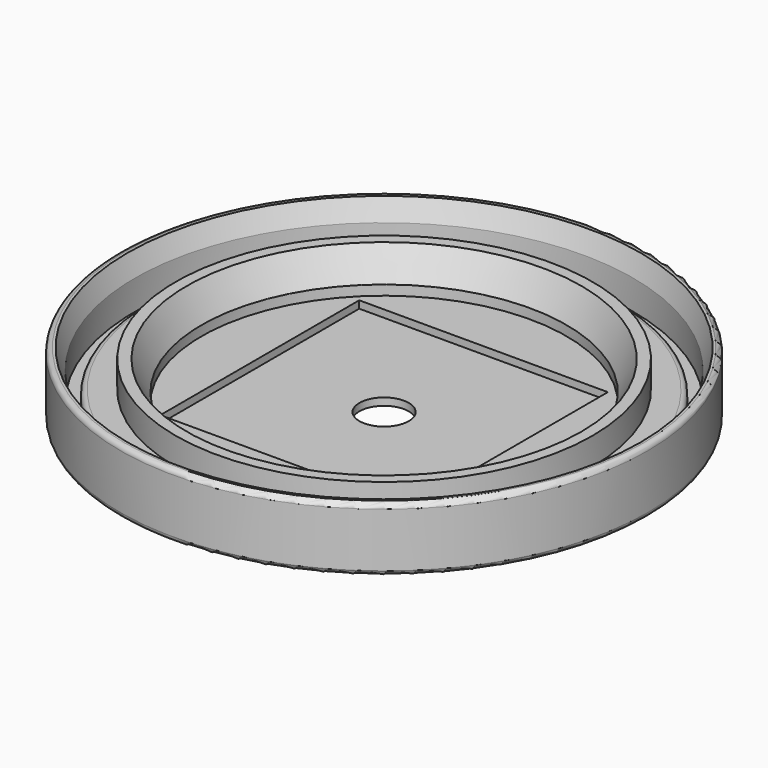
from build123d import *

# Parameters (mm, degrees)
F0_R      = 53.5
F1_DEPTH  = 13
F2_T      = -3
F3_R      = 48
F3_R_2    = 42.25
F3_R_3    = 37
F4_DEPTH  = 2.5
F5_DEPTH  = 8
F6_SIZE2  = 6
F6_SIZE   = 3
F7_SIZE2  = 1.5
F7_SIZE   = 4
F8_R      = 1
F9_R      = 5
F10_DEPTH = 45.7
F11_W     = 50.4
F11_H     = 50.4
F12_DEPTH = 1.5


with BuildPart() as f1:
    # F0 (on Top) → F1 (new body)
    with BuildSketch(Plane.XY):
        Circle(F0_R)
    extrude(amount=F1_DEPTH)

    # F2
    f2_openings = [f1.faces().sort_by_distance(p)[0] for p in [
        (0, 0, 13),
    ]]
    offset(amount=F2_T, openings=f2_openings)

    # F3 (on face) → F4 (join)
    with BuildSketch(Plane.XY.offset(3)):
        Circle(F3_R)
        Circle(F3_R_2, mode=Mode.SUBTRACT)
        Circle(F3_R_2)
        Circle(F3_R_3, mode=Mode.SUBTRACT)
    extrude(amount=F4_DEPTH)

    # F3 (on face) → F5 (join)
    with BuildSketch(Plane.XY.offset(3)):
        Circle(F3_R_2)
        Circle(F3_R_3, mode=Mode.SUBTRACT)
    extrude(amount=F5_DEPTH)

    # F6
    f6_edges = [f1.edges().sort_by_distance(p)[0] for p in [
        (-37, 0, 11),
    ]]
    f6_side = f1.faces().sort_by_distance((-41.05499, 0, 11))[0]
    chamfer(f6_edges, length=F6_SIZE, length2=F6_SIZE2, reference=f6_side)

    # F7
    f7_edges = [f1.edges().sort_by_distance(p)[0] for p in [
        (-50.5, 0, 13),
    ]]
    chamfer(f7_edges, length=F7_SIZE, length2=F7_SIZE2)

    # F8
    f8_edges = [f1.edges().sort_by_distance(p)[0] for p in [
        (-48, 0, 5.5),
        (-53.5, 0, 0),
        (-53.5, 0, 13),
    ]]
    fillet(f8_edges, radius=F8_R)

    # F9 (on face) → F10 (cut, symmetric)
    with BuildSketch(Plane.XY.offset(5.5)):
        Circle(F9_R)
    extrude(amount=F10_DEPTH, both=True, mode=Mode.SUBTRACT)

    # F11 (on face) → F12 (cut)
    with BuildSketch(Plane.XY.offset(3)):
        Rectangle(F11_W, F11_H)
    extrude(amount=-F12_DEPTH, mode=Mode.SUBTRACT)


solid = f1.part
